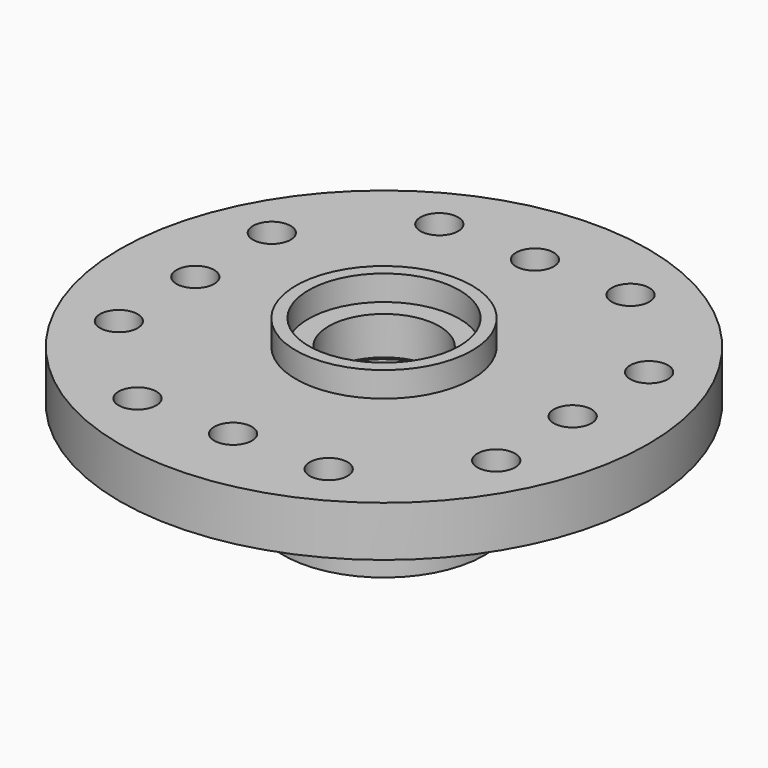
from build123d import *

# Parameters (mm, degrees)
F0_R     = 10.5
F0_R_2   = 0.75
F0_R_3   = 3.5
F0_R_4   = 3
F1_DEPTH = 2
F2_DEPTH = 1
F3_R     = 4
F4_DEPTH = 4
F6_D     = 4.4
F8_D     = 6
F8_DEPTH = 4
F8_TIP   = 1.8025818571


with BuildPart() as f1:
    # F0 (on Top) → F1 (new body)
    with BuildSketch(Plane.XY):
        Circle(F0_R)
        with Locations((-3.8, -7.5)):
            Circle(F0_R_2, mode=Mode.SUBTRACT)
        with Locations((-7.5, -3.8)):
            Circle(F0_R_2, mode=Mode.SUBTRACT)
        with Locations((0, -7.5)):
            Circle(F0_R_2, mode=Mode.SUBTRACT)
        with Locations((3.8, -7.5)):
            Circle(F0_R_2, mode=Mode.SUBTRACT)
        with Locations((7.5, -3.8)):
            Circle(F0_R_2, mode=Mode.SUBTRACT)
        with Locations((-7.5, 0)):
            Circle(F0_R_2, mode=Mode.SUBTRACT)
        with Locations((-7.5, 3.8)):
            Circle(F0_R_2, mode=Mode.SUBTRACT)
        with Locations((-3.8, 7.5)):
            Circle(F0_R_2, mode=Mode.SUBTRACT)
        Circle(F0_R_3, mode=Mode.SUBTRACT)
        with Locations((7.5, 0)):
            Circle(F0_R_2, mode=Mode.SUBTRACT)
        with Locations((7.5, 3.8)):
            Circle(F0_R_2, mode=Mode.SUBTRACT)
        with Locations((0, 7.5)):
            Circle(F0_R_2, mode=Mode.SUBTRACT)
        with Locations((3.8, 7.5)):
            Circle(F0_R_2, mode=Mode.SUBTRACT)
        Circle(F0_R_3)
        Circle(F0_R_4, mode=Mode.SUBTRACT)
        Circle(F0_R_4)
    extrude(amount=-F1_DEPTH)

    # F0 (on Top) → F2 (join)
    with BuildSketch(Plane.XY):
        Circle(F0_R_3)
        Circle(F0_R_4, mode=Mode.SUBTRACT)
    extrude(amount=F2_DEPTH)

    # F3 (on face) → F4 (join)
    with BuildSketch(Plane(origin=(0, 0, -2), x_dir=(1, 0, 0), z_dir=(0, 0, -1))):
        Circle(F3_R)
    extrude(amount=F4_DEPTH)

    # F6 (through all)
    with Locations(Plane.XY):
        with Locations((0, 0)):
            Hole(F6_D / 2)

    # F8
    with Locations(Plane(origin=(0, 0, -6), x_dir=(1, 0, 0), z_dir=(0, 0, -1))):
        with Locations((0, 0)):
            Hole(F8_D / 2, depth=F8_DEPTH)
            with Locations((0, 0, -(F8_DEPTH + F8_TIP / 2))):  # 118° drill point
                Cone(0, F8_D / 2, F8_TIP, mode=Mode.SUBTRACT)


solid = f1.part
